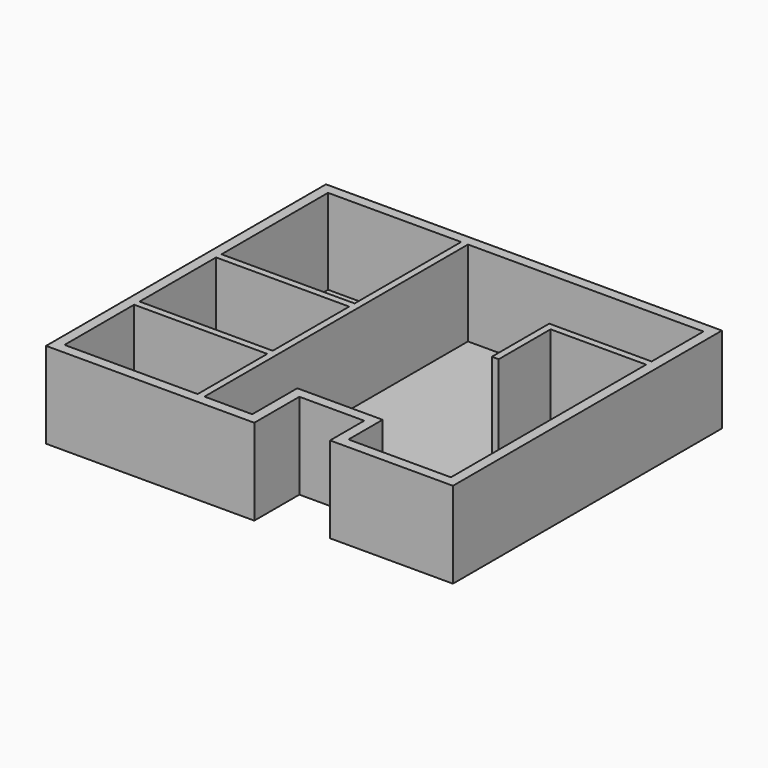
from build123d import *

# Parameters (mm, degrees)
F0_W        = 3900
F0_H        = 200
F1_DEPTH    = 2500
F0_H_2      = 3900
F0_H_3      = 2800
F2_DEPTH    = 25
F3_W        = 1000
F3_H        = 1000
F4_DEPTH    = 1250
F5_T4_DEPTH = 6170.686280177


# Not quite as in the source:
# - a fillet or chamfer that OpenCascade refuses, or shapes differently, is made with other operations: its cross-section is extruded or revolved along the edge and cut away or added


with BuildPart() as f1:
    # F0 (on Top) → F1 (new body)
    with BuildSketch(Plane.XY):
        Polygon((-11300, 8300), (-11300, 2877.939863491), (-11300, -1950), (-5200, -1950), (-5200, -300), (-3300, -300), (-3300, -1550), (300, -1550), (300, 2832.2768892759), (300, 8300), align=None)
        Polygon((-3000, -1250), (-3000, 0), (-5500, 0), (-5500, -1650), (-6900, -1650), (-7100, -1650), (-11000, -1650), (-11000, 0), (-11000, 900), (-11000, 1100), (-11000, 3900), (-11000, 4100), (-11000, 8000), (-7100, 8000), (-6900, 8000), (0, 8000), (0, 6100), (0, 5900), (0, 0), (0, -1250), align=None, mode=Mode.SUBTRACT)
        Polygon((-7100, -1650), (-6900, -1650), (-6900, 8000), (-7100, 8000), (-7100, 4100), (-7100, 3900), (-7100, 1100), (-7100, 900), align=None)
        with Locations((-9050, 4000)):
            Rectangle(F0_W, F0_H)
        with Locations((-9050, 1000)):
            Rectangle(F0_W, F0_H)
        Polygon((-2800, 5900), (0, 5900), (0, 6100), (-3000, 6100), (-3000, 4000), (-2800, 4000), align=None)
    extrude(amount=F1_DEPTH)

    # F0 (on Top) → F2 (join)
    with BuildSketch(Plane.XY):
        Polygon((-11300, 8300), (-11300, 2877.939863491), (-11300, -1950), (-5200, -1950), (-5200, -300), (-3300, -300), (-3300, -1550), (300, -1550), (300, 2832.2768892759), (300, 8300), align=None)
        Polygon((-3000, -1250), (-3000, 0), (-5500, 0), (-5500, -1650), (-6900, -1650), (-7100, -1650), (-11000, -1650), (-11000, 0), (-11000, 900), (-11000, 1100), (-11000, 3900), (-11000, 4100), (-11000, 8000), (-7100, 8000), (-6900, 8000), (0, 8000), (0, 6100), (0, 5900), (0, 0), (0, -1250), align=None, mode=Mode.SUBTRACT)
        with Locations((-9050, 1000)):
            Rectangle(F0_W, F0_H)
        with Locations((-9050, 4000)):
            Rectangle(F0_W, F0_H)
        Polygon((-7100, -1650), (-6900, -1650), (-6900, 8000), (-7100, 8000), (-7100, 4100), (-7100, 3900), (-7100, 1100), (-7100, 900), align=None)
        Polygon((-2800, 5900), (0, 5900), (0, 6100), (-3000, 6100), (-3000, 4000), (-2800, 4000), align=None)
        Polygon((-5500, 0), (-3000, 0), (-3000, -1250), (0, -1250), (0, 0), (0, 5900), (-2800, 5900), (-2800, 4000), (-3000, 4000), (-3000, 6100), (0, 6100), (0, 8000), (-6900, 8000), (-6900, -1650), (-5500, -1650), align=None)
        with Locations((-9050, 6050)):
            Rectangle(F0_W, F0_H_2)
        with Locations((-9050, 2500)):
            Rectangle(F0_W, F0_H_3)
        Polygon((-11000, -1650), (-7100, -1650), (-7100, 900), (-11000, 900), (-11000, 0), align=None)
    extrude(amount=-F2_DEPTH)

    # F3 (on face) → F4 (join)
    with BuildSketch(Plane.XY):
        with Locations((-500, 3500)):
            Rectangle(F3_W, F3_H)
        Polygon((-3000, 3000), (-1000, 3000), (-1000, 4000), (-2800, 4000), (-3000, 4000), align=None)
    extrude(amount=F4_DEPTH)

    # F5: chamfer of 1250 x 2000 on 1 edges, made by hand


with BuildPart() as f5_tool2:
    # F5_s3 → F5_t4 (new body)
    with BuildSketch(Plane.XZ.offset(-4000)):
        Polygon((-1000, 1250), (-3000, 0), (-3000, 1250), align=None)
    extrude(amount=F5_T4_DEPTH)

    split(bisect_by=Plane.XZ, keep=Keep.BOTTOM)


with BuildPart() as f1_1:
    add(f1.part)

    # F5_t1: cut F5_tool2
    add(f5_tool2.part, mode=Mode.SUBTRACT)


solid = f1_1.part
